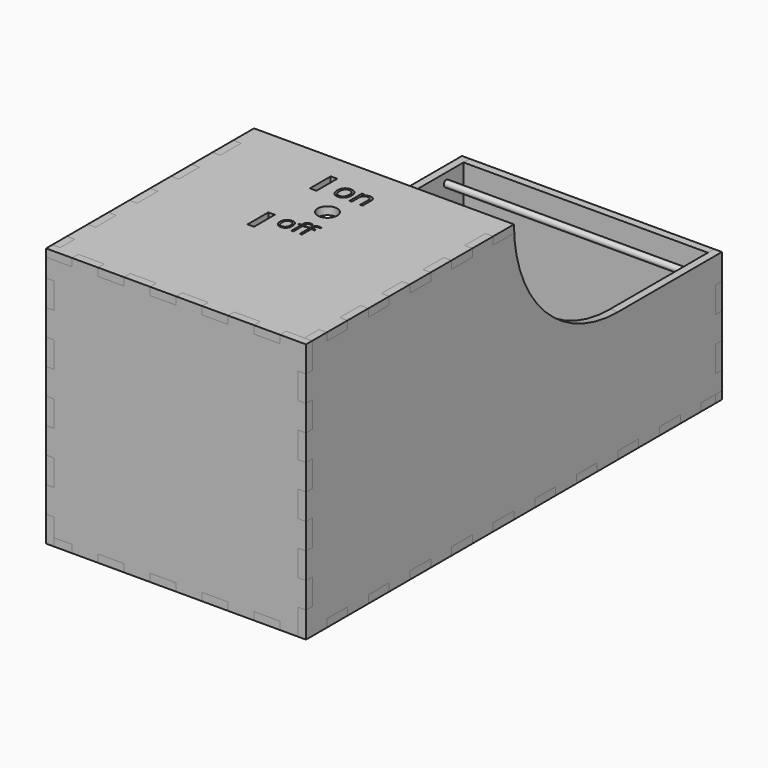
from build123d import *

# Parameters (mm, degrees)
F1_DEPTH        = 3
F2_DEPTH        = 3
F6_DEPTH        = 3
F8_START        = -197
F8_DEPTH        = 3
F9_START        = -197
F9_DEPTH        = 3
F12_W           = 100
F12_H           = 100
F13_DEPTH       = 3
F14_DEPTH       = 3
F15_START       = -97
F15_DEPTH       = 3
F23_R           = 1.25
F24_DEPTH       = 100
F25_R           = 3.75
F26_DEPTH       = 25
F27_W           = 2.5
F27_H           = 10
F28_DEPTH       = 5
F29_TEXT_SIZE   = 9.6153519634
F29_TEXT_SIZE_2 = 11.2636946142
F30_DEPTH       = 5


# Not quite as in the source:
# - Text() gives the source's letters only with a copy of the font that has no kerning and outlines rounded to 1/6400 em; it was checked with that copy


with BuildPart() as f1:
    # F0 (on Right) → F1 (new body)
    with BuildSketch(Plane.YZ):
        with BuildLine():
            Line((10, 0), (3, 0))
            Line((3, 0), (3, -10))
            Line((3, -10), (0, -10))
            Line((0, -10), (0, -20))
            Line((0, -20), (3, -20))
            Line((3, -20), (3, -30))
            Line((3, -30), (0, -30))
            Line((0, -30), (0, -40))
            Line((0, -40), (3, -40))
            Line((3, -40), (3, -50))
            Line((3, -50), (0, -50))
            Line((0, -50), (0, -60))
            Line((0, -60), (3, -60))
            Line((3, -60), (3, -70))
            Line((3, -70), (0, -70))
            Line((0, -70), (0, -80))
            Line((0, -80), (3, -80))
            Line((3, -80), (3, -90))
            Line((3, -90), (0, -90))
            Line((0, -90), (0, -100))
            Line((0, -100), (10, -100))
            Line((10, -100), (10, -97))
            Line((10, -97), (20, -97))
            Line((20, -97), (20, -100))
            Line((20, -100), (30, -100))
            Line((30, -100), (30, -97))
            Line((30, -97), (40, -97))
            Line((40, -97), (40, -100))
            Line((40, -100), (50, -100))
            Line((50, -100), (50, -97))
            Line((50, -97), (60, -97))
            Line((60, -97), (60, -100))
            Line((60, -100), (70, -100))
            Line((70, -100), (70, -97))
            Line((70, -97), (80, -97))
            Line((80, -97), (80, -100))
            Line((80, -100), (90, -100))
            Line((90, -100), (90, -97))
            Line((90, -97), (100, -97))
            Line((100, -97), (100, -100))
            Line((100, -100), (110, -100))
            Line((110, -100), (110, -97))
            Line((110, -97), (120, -97))
            Line((120, -97), (120, -100))
            Line((120, -100), (130, -100))
            Line((130, -100), (130, -97))
            Line((130, -97), (140, -97))
            Line((140, -97), (140, -100))
            Line((140, -100), (150, -100))
            Line((150, -100), (150, -97))
            Line((150, -97), (160, -97))
            Line((160, -97), (160, -100))
            Line((160, -100), (170, -100))
            Line((170, -100), (170, -97))
            Line((170, -97), (180, -97))
            Line((180, -97), (180, -100))
            Line((180, -100), (190, -100))
            Line((190, -100), (190, -97))
            Line((190, -97), (200, -97))
            Line((200, -97), (200, -90))
            Line((200, -90), (197, -90))
            Line((197, -90), (197, -80))
            Line((197, -80), (200, -80))
            Line((200, -80), (200, -70))
            Line((200, -70), (197, -70))
            Line((197, -70), (197, -60))
            Line((197, -60), (200, -60))
            Line((200, -60), (200, -50))
            Line((200, -50), (197, -50))
            Line((197, -50), (150, -50))
            ThreePointArc((150, -50), (114.6446609407, -35.3553390593), (100, 0))
            Line((100, 0), (100, -3))
            Line((100, -3), (90, -3))
            Line((90, -3), (90, 0))
            Line((90, 0), (80, 0))
            Line((80, 0), (80, -3))
            Line((80, -3), (70, -3))
            Line((70, -3), (70, 0))
            Line((70, 0), (60, 0))
            Line((60, 0), (60, -3))
            Line((60, -3), (50, -3))
            Line((50, -3), (50, 0))
            Line((50, 0), (40, 0))
            Line((40, 0), (40, -3))
            Line((40, -3), (30, -3))
            Line((30, -3), (30, 0))
            Line((30, 0), (20, 0))
            Line((20, 0), (20, -3))
            Line((20, -3), (10, -3))
            Line((10, -3), (10, 0))
        make_face()
    extrude(amount=F1_DEPTH)


with BuildPart() as f2:
    # F0 (on Right) → F2 (new body)
    with BuildSketch(Plane.YZ):
        with BuildLine():
            Line((110, 0), (100, 0))
            ThreePointArc((100, 0), (114.6446609407, -35.3553390593), (150, -50))
            Line((150, -50), (197, -50))
            Line((197, -50), (197, -40))
            Line((197, -40), (200, -40))
            Line((200, -40), (200, -30))
            Line((200, -30), (197, -30))
            Line((197, -30), (197, -20))
            Line((197, -20), (200, -20))
            Line((200, -20), (200, -10))
            Line((200, -10), (197, -10))
            Line((197, -10), (197, -3))
            Line((197, -3), (190, -3))
            Line((190, -3), (190, 0))
            Line((190, 0), (180, 0))
            Line((180, 0), (180, -3))
            Line((180, -3), (170, -3))
            Line((170, -3), (170, 0))
            Line((170, 0), (160, 0))
            Line((160, 0), (160, -3))
            Line((160, -3), (150, -3))
            Line((150, -3), (150, 0))
            Line((150, 0), (140, 0))
            Line((140, 0), (140, -3))
            Line((140, -3), (130, -3))
            Line((130, -3), (130, 0))
            Line((130, 0), (120, 0))
            Line((120, 0), (120, -3))
            Line((120, -3), (110, -3))
            Line((110, -3), (110, 0))
        make_face()
    extrude(amount=F2_DEPTH)


with BuildPart() as f4_1:
    # F4: copy of F1
    add(f1.part.moved(Location((-97, 0, 0))))


with BuildPart() as f5_1:
    # F5: copy of F2
    add(f2.part.moved(Location((-97, 0, 0))))


with BuildPart() as f6:
    # F3 (on Front) → F6 (new body)
    with BuildSketch(Plane.XZ):
        Polygon((3, -50), (3, 0), (-7, 0), (-7, -3), (-17, -3), (-17, 0), (-27, 0), (-27, -3), (-37, -3), (-37, 0), (-47, 0), (-47, -3), (-57, -3), (-57, 0), (-67, 0), (-67, -3), (-77, -3), (-77, 0), (-87, 0), (-87, -3), (-97, -3), (-97, -50), align=None)
        Polygon((3, -100), (3, -50), (-97, -50), (-97, -97), (-87, -97), (-87, -100), (-77, -100), (-77, -97), (-67, -97), (-67, -100), (-57, -100), (-57, -97), (-47, -97), (-47, -100), (-37, -100), (-37, -97), (-27, -97), (-27, -100), (-17, -100), (-17, -97), (-7, -97), (-7, -100), align=None)
    extrude(amount=-F6_DEPTH)

    # F7: cut F4_1, F1
    add(f4_1.part, mode=Mode.SUBTRACT)
    add(f1.part, mode=Mode.SUBTRACT)


with BuildPart() as f8:
    # F3 (on Front) → F8 (new body)
    with BuildSketch(Plane.XZ.offset(F8_START)):
        Polygon((3, -100), (3, -50), (-97, -50), (-97, -97), (-87, -97), (-87, -100), (-77, -100), (-77, -97), (-67, -97), (-67, -100), (-57, -100), (-57, -97), (-47, -97), (-47, -100), (-37, -100), (-37, -97), (-27, -97), (-27, -100), (-17, -100), (-17, -97), (-7, -97), (-7, -100), align=None)
    extrude(amount=-F8_DEPTH)

    # F11: cut F1, F4_1
    add(f1.part, mode=Mode.SUBTRACT)
    add(f4_1.part, mode=Mode.SUBTRACT)


with BuildPart() as f9:
    # F3 (on Front) → F9 (new body)
    with BuildSketch(Plane.XZ.offset(F9_START)):
        Polygon((3, -50), (3, 0), (-7, 0), (-7, -3), (-17, -3), (-17, 0), (-27, 0), (-27, -3), (-37, -3), (-37, 0), (-47, 0), (-47, -3), (-57, -3), (-57, 0), (-67, 0), (-67, -3), (-77, -3), (-77, 0), (-87, 0), (-87, -3), (-97, -3), (-97, -50), align=None)
    extrude(amount=-F9_DEPTH)

    # F10: cut F2, F5_1
    add(f2.part, mode=Mode.SUBTRACT)
    add(f5_1.part, mode=Mode.SUBTRACT)


with BuildPart() as f13:
    # F12 (on Top) → F13 (new body)
    with BuildSketch(Plane.XY):
        with Locations((-47, 50)):
            Rectangle(F12_W, F12_H)
    extrude(amount=-F13_DEPTH)

    # F17: cut F6, F1, F4_1
    add(f6.part, mode=Mode.SUBTRACT)
    add(f1.part, mode=Mode.SUBTRACT)
    add(f4_1.part, mode=Mode.SUBTRACT)

    # F25 (on face) → F26 (cut)
    with BuildSketch(Plane.XY):
        with Locations((-45.75, 71.25)):
            Circle(F25_R)
    extrude(amount=-F26_DEPTH, mode=Mode.SUBTRACT)

    # F27 (on face) → F28 (cut)
    with BuildSketch(Plane.XY):
        with Locations((-58.25, 85)):
            Rectangle(F27_W, F27_H)
        with Locations((-58.25, 55)):
            Rectangle(F27_W, F27_H)
    extrude(amount=-F28_DEPTH, mode=Mode.SUBTRACT)

    # F29 (on face) → F30 (cut)
    with BuildSketch(Plane.XY):
        with Locations((-53.5263828933, 54.982803762)):
            Text('off', F29_TEXT_SIZE, font='Open Sans', text_align=(TextAlign.LEFT, TextAlign.BOTTOM))
        with Locations((-52.9329776764, 81.0926109552)):
            Text('on', F29_TEXT_SIZE_2, font='Open Sans', text_align=(TextAlign.LEFT, TextAlign.BOTTOM))
    extrude(amount=-F30_DEPTH, mode=Mode.SUBTRACT)


with BuildPart() as f14:
    # F12 (on Top) → F14 (new body)
    with BuildSketch(Plane.XY):
        with Locations((-47, 150)):
            Rectangle(F12_W, F12_H)
    extrude(amount=-F14_DEPTH)

    # F18: cut F2, F9, F5_1
    add(f2.part, mode=Mode.SUBTRACT)
    add(f9.part, mode=Mode.SUBTRACT)
    add(f5_1.part, mode=Mode.SUBTRACT)


with BuildPart() as f15:
    # F12 (on Top) → F15 (new body)
    with BuildSketch(Plane.XY.offset(F15_START)):
        with Locations((-47, 150)):
            Rectangle(F12_W, F12_H)
        with Locations((-47, 50)):
            Rectangle(F12_W, F12_H)
    extrude(amount=-F15_DEPTH)

    # F16: cut F6, F1, F8, F4_1
    add(f6.part, mode=Mode.SUBTRACT)
    add(f1.part, mode=Mode.SUBTRACT)
    add(f8.part, mode=Mode.SUBTRACT)
    add(f4_1.part, mode=Mode.SUBTRACT)


with BuildPart() as f1_1:
    add(f1.part)

    # F23 (on face) → F24 (join)
    with BuildSketch(Plane.YZ.offset(3)):
        with Locations((188.75, -53.75)):
            Circle(F23_R)
    extrude(amount=-F24_DEPTH)


solid = Compound([f4_1.part, f6.part, f8.part, f13.part, f15.part, f1_1.part])
